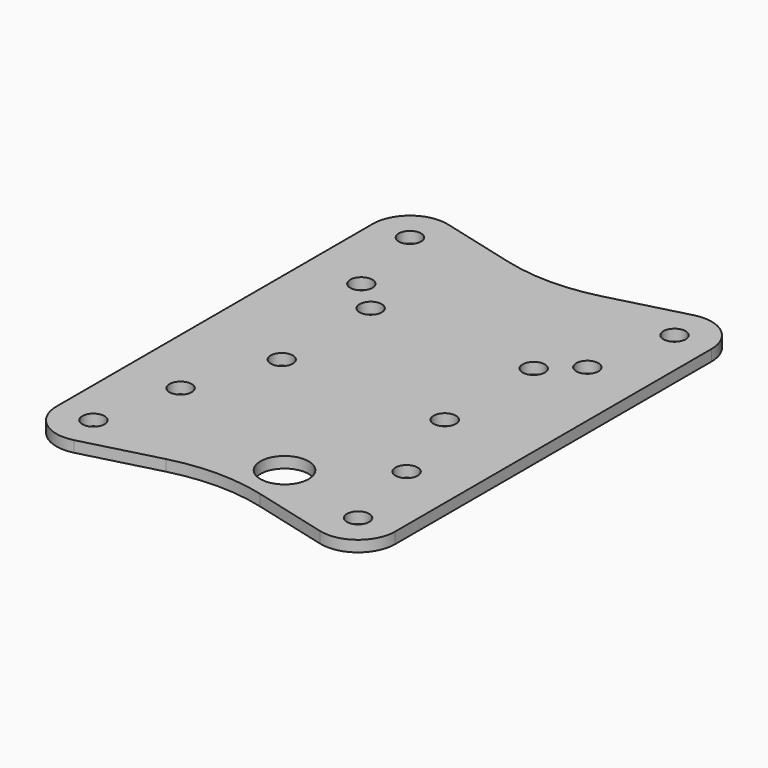
from build123d import *

# Parameters (mm, degrees)
F0_R     = 1.5
F0_R_2   = 3.25
F1_DEPTH = 1.5


# Not quite as in the source:
# - ends of sketch curves that miss each other by under 0.0002 mm in the source are joined


with BuildPart() as f1:
    # F0 (on Top) → F1 (new body)
    with BuildSketch(Plane.XY):
        with BuildLine():
            ThreePointArc((6.3250610024, 28.8463679906), (-4.837e-07, 28.033009), (-6.3250619384, 28.8463682354))
            Line((-6.3250619384, 28.8463682354), (-16.589434, 31.530609))
            ThreePointArc((-16.589434, 31.530609), (-20.910174001, 30.6508727545), (-22.854447, 26.693281))
            Line((-22.854447, 26.693281), (-22.854447, -26.693281))
            ThreePointArc((-22.854447, -26.693281), (-20.910174001, -30.6508727545), (-16.5894340018, -31.5306089933))
            Line((-16.5894340018, -31.5306089933), (-6.325062, -28.846368))
            ThreePointArc((-6.325062, -28.846368), (-4.837e-07, -28.033009), (6.3250610024, -28.8463679906))
            Line((6.3250610024, -28.8463679906), (16.589434, -31.530609))
            ThreePointArc((16.589434, -31.530609), (20.9101733838, -30.6508724589), (22.854446, -26.693281))
            Line((22.854446, -26.693281), (22.854446, 26.693281))
            ThreePointArc((22.854446, 26.693281), (20.9101733838, 30.6508724589), (16.5894339378, 31.530609238))
            Line((16.5894339378, 31.530609238), (6.3250610024, 28.8463679906))
        make_face()
        with Locations((-17.854447, -26.693281)):
            Circle(F0_R, mode=Mode.SUBTRACT)
        with Locations((-15.25, -15.25)):
            Circle(F0_R, mode=Mode.SUBTRACT)
        with Locations((-11, -3.5)):
            Circle(F0_R, mode=Mode.SUBTRACT)
        with Locations((5, -23.033009)):
            Circle(F0_R_2, mode=Mode.SUBTRACT)
        with Locations((17.854446, -26.693281)):
            Circle(F0_R, mode=Mode.SUBTRACT)
        with Locations((11, -3.5)):
            Circle(F0_R, mode=Mode.SUBTRACT)
        with Locations((15.25, -15.25)):
            Circle(F0_R, mode=Mode.SUBTRACT)
        with Locations((-15.25, 15.25)):
            Circle(F0_R, mode=Mode.SUBTRACT)
        with Locations((-11, 11.5)):
            Circle(F0_R, mode=Mode.SUBTRACT)
        with Locations((-17.854447, 26.693281)):
            Circle(F0_R, mode=Mode.SUBTRACT)
        with Locations((11, 11.5)):
            Circle(F0_R, mode=Mode.SUBTRACT)
        with Locations((15.25, 15.25)):
            Circle(F0_R, mode=Mode.SUBTRACT)
        with Locations((17.854446, 26.693281)):
            Circle(F0_R, mode=Mode.SUBTRACT)
    extrude(amount=F1_DEPTH)


solid = f1.part
